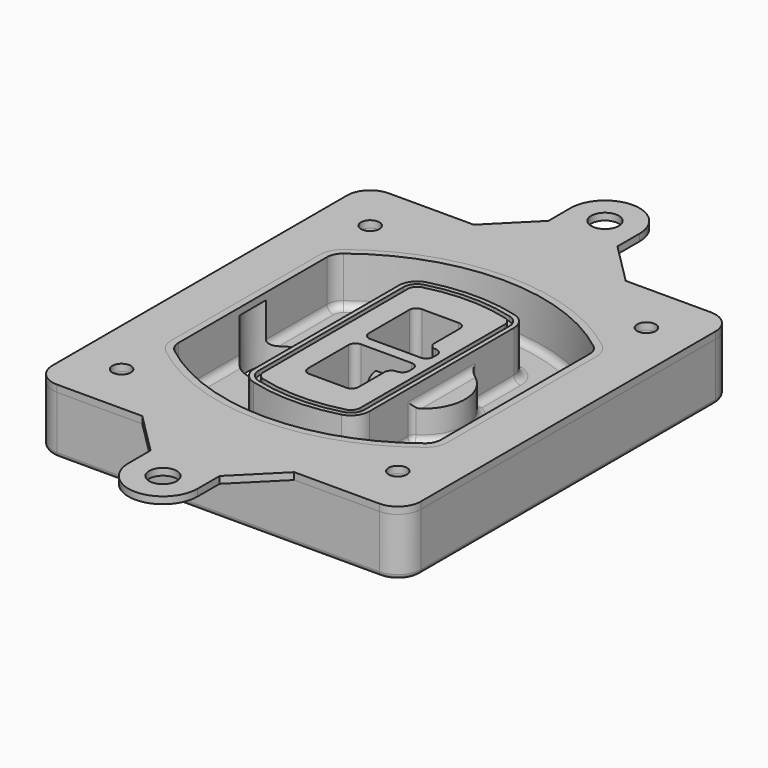
from build123d import *

# Parameters (mm, degrees)
F0_R      = 4
F1_DEPTH  = 25
F2_DEPTH  = 3
F3_DEPTH  = 18
F5_DEPTH  = 21
F6_DEPTH  = 2
F8_DEPTH  = 20
F9_DEPTH  = 16
F10_DEPTH = 25
F7_R      = 6
F7_R_2    = 4
F11_DEPTH = 6
F13_DEPTH = 9
F14_R     = 3
F15_R     = 2
F16_R     = 4
F17_DEPTH = 3
F18_D     = 12


with BuildPart() as f1:
    # F0 (on Top) → F1 (new body)
    with BuildSketch(Plane.XY):
        with BuildLine():
            ThreePointArc((-80, -80), (-77.0710678119, -87.0710678119), (-70, -90))
            Line((-70, -90), (70, -90))
            ThreePointArc((70, -90), (77.0710678119, -87.0710678119), (80, -80))
            Line((80, -80), (80, 80))
            ThreePointArc((80, 80), (77.0710678119, 87.0710678119), (70, 90))
            Line((70, 90), (-70, 90))
            ThreePointArc((-70, 90), (-77.0710678119, 87.0710678119), (-80, 80))
            Line((-80, 80), (-80, -80))
        make_face()
        with Locations((-60, -67.5)):
            Circle(F0_R, mode=Mode.SUBTRACT)
        with Locations((60, -67.5)):
            Circle(F0_R, mode=Mode.SUBTRACT)
        with Locations((-60, 67.5)):
            Circle(F0_R, mode=Mode.SUBTRACT)
        with BuildLine():
            ThreePointArc((-64, 40.2934422872), (-62.5820384798, 46.4328484224), (-58.6153846154, 51.3286200352))
            ThreePointArc((-58.6153846154, 51.3286200352), (0, 71.5), (58.6153846154, 51.3286200352))
            ThreePointArc((58.6153846154, 51.3286200352), (62.5820384798, 46.4328484224), (64, 40.2934422872))
            Line((64, 40.2934422872), (64, -40.2934422872))
            ThreePointArc((64, -40.2934422872), (62.5820384798, -46.4328484224), (58.6153846154, -51.3286200352))
            ThreePointArc((58.6153846154, -51.3286200352), (0, -71.5), (-58.6153846154, -51.3286200352))
            ThreePointArc((-58.6153846154, -51.3286200352), (-62.5820384798, -46.4328484224), (-64, -40.2934422872))
            Line((-64, -40.2934422872), (-64, 40.2934422872))
        make_face(mode=Mode.SUBTRACT)
        with Locations((60, 67.5)):
            Circle(F0_R, mode=Mode.SUBTRACT)
        with BuildLine():
            ThreePointArc((58.6153846154, 51.3286200352), (0, 71.5), (-58.6153846154, 51.3286200352))
            ThreePointArc((-58.6153846154, 51.3286200352), (-62.5820384798, 46.4328484224), (-64, 40.2934422872))
            Line((-64, 40.2934422872), (-64, -40.2934422872))
            ThreePointArc((-64, -40.2934422872), (-62.5820384798, -46.4328484224), (-58.6153846154, -51.3286200352))
            ThreePointArc((-58.6153846154, -51.3286200352), (0, -71.5), (58.6153846154, -51.3286200352))
            ThreePointArc((58.6153846154, -51.3286200352), (62.5820384798, -46.4328484224), (64, -40.2934422872))
            Line((64, -40.2934422872), (64, 40.2934422872))
            ThreePointArc((64, 40.2934422872), (62.5820384798, 46.4328484224), (58.6153846154, 51.3286200352))
        make_face()
        with BuildLine():
            Line((-60, -40.2934422872), (-60, 40.2934422872))
            ThreePointArc((-60, 40.2934422872), (-58.9871703427, 44.6787323838), (-56.1538461538, 48.1757121072))
            ThreePointArc((-56.1538461538, 48.1757121072), (0, 67.5), (56.1538461538, 48.1757121072))
            ThreePointArc((56.1538461538, 48.1757121072), (58.9871703427, 44.6787323838), (60, 40.2934422872))
            Line((60, 40.2934422872), (60, -40.2934422872))
            ThreePointArc((60, -40.2934422872), (58.9871703427, -44.6787323838), (56.1538461538, -48.1757121072))
            ThreePointArc((56.1538461538, -48.1757121072), (0, -67.5), (-56.1538461538, -48.1757121072))
            ThreePointArc((-56.1538461538, -48.1757121072), (-58.9871703427, -44.6787323838), (-60, -40.2934422872))
        make_face(mode=Mode.SUBTRACT)
        with BuildLine():
            ThreePointArc((-56.1538461538, 48.1757121072), (-58.9871703427, 44.6787323838), (-60, 40.2934422872))
            Line((-60, 40.2934422872), (-60, -40.2934422872))
            ThreePointArc((-60, -40.2934422872), (-58.9871703427, -44.6787323838), (-56.1538461538, -48.1757121072))
            ThreePointArc((-56.1538461538, -48.1757121072), (0, -67.5), (56.1538461538, -48.1757121072))
            ThreePointArc((56.1538461538, -48.1757121072), (58.9871703427, -44.6787323838), (60, -40.2934422872))
            Line((60, -40.2934422872), (60, 40.2934422872))
            ThreePointArc((60, 40.2934422872), (58.9871703427, 44.6787323838), (56.1538461538, 48.1757121072))
            ThreePointArc((56.1538461538, 48.1757121072), (0, 67.5), (-56.1538461538, 48.1757121072))
        make_face()
        with BuildLine():
            ThreePointArc((54.3076923077, 45.8110311612), (56.2910192399, 43.3631453548), (57, 40.2934422872))
            Line((57, 40.2934422872), (57, -40.2934422872))
            ThreePointArc((57, -40.2934422872), (56.2910192399, -43.3631453548), (54.3076923077, -45.8110311612))
            ThreePointArc((54.3076923077, -45.8110311612), (0, -64.5), (-54.3076923077, -45.8110311612))
            ThreePointArc((-54.3076923077, -45.8110311612), (-56.2910192399, -43.3631453548), (-57, -40.2934422872))
            Line((-57, -40.2934422872), (-57, 40.2934422872))
            ThreePointArc((-57, 40.2934422872), (-56.2910192399, 43.3631453548), (-54.3076923077, 45.8110311612))
            ThreePointArc((-54.3076923077, 45.8110311612), (0, 64.5), (54.3076923077, 45.8110311612))
        make_face(mode=Mode.SUBTRACT)
        with BuildLine():
            Line((57, -40.2934422872), (57, 40.2934422872))
            ThreePointArc((57, 40.2934422872), (56.2910192399, 43.3631453548), (54.3076923077, 45.8110311612))
            ThreePointArc((54.3076923077, 45.8110311612), (0, 64.5), (-54.3076923077, 45.8110311612))
            ThreePointArc((-54.3076923077, 45.8110311612), (-56.2910192399, 43.3631453548), (-57, 40.2934422872))
            Line((-57, 40.2934422872), (-57, -40.2934422872))
            ThreePointArc((-57, -40.2934422872), (-56.2910192399, -43.3631453548), (-54.3076923077, -45.8110311612))
            ThreePointArc((-54.3076923077, -45.8110311612), (0, -64.5), (54.3076923077, -45.8110311612))
            ThreePointArc((54.3076923077, -45.8110311612), (56.2910192399, -43.3631453548), (57, -40.2934422872))
        make_face()
    extrude(amount=-F1_DEPTH)

    # F0 (on Top) → F2 (join)
    with BuildSketch(Plane.XY):
        with BuildLine():
            ThreePointArc((-56.1538461538, 48.1757121072), (-58.9871703427, 44.6787323838), (-60, 40.2934422872))
            Line((-60, 40.2934422872), (-60, -40.2934422872))
            ThreePointArc((-60, -40.2934422872), (-58.9871703427, -44.6787323838), (-56.1538461538, -48.1757121072))
            ThreePointArc((-56.1538461538, -48.1757121072), (0, -67.5), (56.1538461538, -48.1757121072))
            ThreePointArc((56.1538461538, -48.1757121072), (58.9871703427, -44.6787323838), (60, -40.2934422872))
            Line((60, -40.2934422872), (60, 40.2934422872))
            ThreePointArc((60, 40.2934422872), (58.9871703427, 44.6787323838), (56.1538461538, 48.1757121072))
            ThreePointArc((56.1538461538, 48.1757121072), (0, 67.5), (-56.1538461538, 48.1757121072))
        make_face()
        with BuildLine():
            ThreePointArc((54.3076923077, 45.8110311612), (56.2910192399, 43.3631453548), (57, 40.2934422872))
            Line((57, 40.2934422872), (57, -40.2934422872))
            ThreePointArc((57, -40.2934422872), (56.2910192399, -43.3631453548), (54.3076923077, -45.8110311612))
            ThreePointArc((54.3076923077, -45.8110311612), (0, -64.5), (-54.3076923077, -45.8110311612))
            ThreePointArc((-54.3076923077, -45.8110311612), (-56.2910192399, -43.3631453548), (-57, -40.2934422872))
            Line((-57, -40.2934422872), (-57, 40.2934422872))
            ThreePointArc((-57, 40.2934422872), (-56.2910192399, 43.3631453548), (-54.3076923077, 45.8110311612))
            ThreePointArc((-54.3076923077, 45.8110311612), (0, 64.5), (54.3076923077, 45.8110311612))
        make_face(mode=Mode.SUBTRACT)
    extrude(amount=F2_DEPTH)

    # F0 (on Top) → F3 (cut)
    with BuildSketch(Plane.XY):
        with BuildLine():
            Line((57, -40.2934422872), (57, 40.2934422872))
            ThreePointArc((57, 40.2934422872), (56.2910192399, 43.3631453548), (54.3076923077, 45.8110311612))
            ThreePointArc((54.3076923077, 45.8110311612), (0, 64.5), (-54.3076923077, 45.8110311612))
            ThreePointArc((-54.3076923077, 45.8110311612), (-56.2910192399, 43.3631453548), (-57, 40.2934422872))
            Line((-57, 40.2934422872), (-57, -40.2934422872))
            ThreePointArc((-57, -40.2934422872), (-56.2910192399, -43.3631453548), (-54.3076923077, -45.8110311612))
            ThreePointArc((-54.3076923077, -45.8110311612), (0, -64.5), (54.3076923077, -45.8110311612))
            ThreePointArc((54.3076923077, -45.8110311612), (56.2910192399, -43.3631453548), (57, -40.2934422872))
        make_face()
    extrude(amount=-F3_DEPTH, mode=Mode.SUBTRACT)

    # F4 (on face) → F5 (join, through all)
    with BuildSketch(Plane.XY.offset(3)):
        with BuildLine():
            ThreePointArc((-25, -39.2465276821), (-23.3511545998, -44.1109737193), (-19.0842911877, -46.9702398883))
            ThreePointArc((-19.0842911877, -46.9702398883), (0, -49.5), (19.0842911877, -46.9702398883))
            ThreePointArc((19.0842911877, -46.9702398883), (23.3511545998, -44.1109737193), (25, -39.2465276821))
            Line((25, -39.2465276821), (25, 39.2465276821))
            ThreePointArc((25, 39.2465276821), (23.3511545998, 44.1109737193), (19.0842911877, 46.9702398883))
            ThreePointArc((19.0842911877, 46.9702398883), (0, 49.5), (-19.0842911877, 46.9702398883))
            ThreePointArc((-19.0842911877, 46.9702398883), (-23.3511545998, 44.1109737193), (-25, 39.2465276821))
            Line((-25, 39.2465276821), (-25, -39.2465276821))
        make_face()
        with BuildLine():
            ThreePointArc((18.5632183908, 45.0393118368), (21.7633659499, 42.89486221), (23, 39.2465276821))
            Line((23, 39.2465276821), (23, -39.2465276821))
            ThreePointArc((23, -39.2465276821), (21.7633659499, -42.89486221), (18.5632183908, -45.0393118368))
            ThreePointArc((18.5632183908, -45.0393118368), (0, -47.5), (-18.5632183908, -45.0393118368))
            ThreePointArc((-18.5632183908, -45.0393118368), (-21.7633659499, -42.89486221), (-23, -39.2465276821))
            Line((-23, -39.2465276821), (-23, 39.2465276821))
            ThreePointArc((-23, 39.2465276821), (-21.7633659499, 42.89486221), (-18.5632183908, 45.0393118368))
            ThreePointArc((-18.5632183908, 45.0393118368), (0, 47.5), (18.5632183908, 45.0393118368))
        make_face(mode=Mode.SUBTRACT)
        with BuildLine():
            Line((23, -39.2465276821), (23, 39.2465276821))
            ThreePointArc((23, 39.2465276821), (21.7633659499, 42.89486221), (18.5632183908, 45.0393118368))
            ThreePointArc((18.5632183908, 45.0393118368), (0, 47.5), (-18.5632183908, 45.0393118368))
            ThreePointArc((-18.5632183908, 45.0393118368), (-21.7633659499, 42.89486221), (-23, 39.2465276821))
            Line((-23, 39.2465276821), (-23, -39.2465276821))
            ThreePointArc((-23, -39.2465276821), (-21.7633659499, -42.89486221), (-18.5632183908, -45.0393118368))
            ThreePointArc((-18.5632183908, -45.0393118368), (0, -47.5), (18.5632183908, -45.0393118368))
            ThreePointArc((18.5632183908, -45.0393118368), (21.7633659499, -42.89486221), (23, -39.2465276821))
        make_face()
        with BuildLine():
            ThreePointArc((18.0421455939, 43.1083837852), (20.1755772999, 41.6787507007), (21, 39.2465276821))
            Line((21, 39.2465276821), (21, -39.2465276821))
            ThreePointArc((21, -39.2465276821), (20.1755772999, -41.6787507007), (18.0421455939, -43.1083837852))
            ThreePointArc((18.0421455939, -43.1083837852), (0, -45.5), (-18.0421455939, -43.1083837852))
            ThreePointArc((-18.0421455939, -43.1083837852), (-20.1755772999, -41.6787507007), (-21, -39.2465276821))
            Line((-21, -39.2465276821), (-21, 39.2465276821))
            ThreePointArc((-21, 39.2465276821), (-20.1755772999, 41.6787507007), (-18.0421455939, 43.1083837852))
            ThreePointArc((-18.0421455939, 43.1083837852), (0, 45.5), (18.0421455939, 43.1083837852))
        make_face(mode=Mode.SUBTRACT)
        with BuildLine():
            Line((21, -39.2465276821), (21, 39.2465276821))
            ThreePointArc((21, 39.2465276821), (20.1755772999, 41.6787507007), (18.0421455939, 43.1083837852))
            ThreePointArc((18.0421455939, 43.1083837852), (0, 45.5), (-18.0421455939, 43.1083837852))
            ThreePointArc((-18.0421455939, 43.1083837852), (-20.1755772999, 41.6787507007), (-21, 39.2465276821))
            Line((-21, 39.2465276821), (-21, -39.2465276821))
            ThreePointArc((-21, -39.2465276821), (-20.1755772999, -41.6787507007), (-18.0421455939, -43.1083837852))
            ThreePointArc((-18.0421455939, -43.1083837852), (0, -45.5), (18.0421455939, -43.1083837852))
            ThreePointArc((18.0421455939, -43.1083837852), (20.1755772999, -41.6787507007), (21, -39.2465276821))
        make_face()
        with BuildLine():
            Line((-8, -2.5), (14, -2.5))
            ThreePointArc((14, -2.5), (16.1213203436, -3.3786796564), (17, -5.5))
            Line((17, -5.5), (17, -7.5))
            ThreePointArc((17, -7.5), (16.1213203436, -9.6213203436), (14, -10.5))
            ThreePointArc((14, -10.5), (11.8786796564, -11.3786796564), (11, -13.5))
            Line((11, -13.5), (11, -27.5))
            ThreePointArc((11, -27.5), (10.1213203436, -29.6213203436), (8, -30.5))
            Line((8, -30.5), (-8, -30.5))
            ThreePointArc((-8, -30.5), (-10.1213203436, -29.6213203436), (-11, -27.5))
            Line((-11, -27.5), (-11, -5.5))
            ThreePointArc((-11, -5.5), (-10.1213203436, -3.3786796564), (-8, -2.5))
        make_face(mode=Mode.SUBTRACT)
        with BuildLine():
            ThreePointArc((-8, 2.5), (-10.1213203436, 3.3786796564), (-11, 5.5))
            Line((-11, 5.5), (-11, 27.5))
            ThreePointArc((-11, 27.5), (-10.1213203436, 29.6213203436), (-8, 30.5))
            Line((-8, 30.5), (8, 30.5))
            ThreePointArc((8, 30.5), (10.1213203436, 29.6213203436), (11, 27.5))
            Line((11, 27.5), (11, 13.5))
            ThreePointArc((11, 13.5), (11.8786796564, 11.3786796564), (14, 10.5))
            ThreePointArc((14, 10.5), (16.1213203436, 9.6213203436), (17, 7.5))
            Line((17, 7.5), (17, 5.5))
            ThreePointArc((17, 5.5), (16.1213203436, 3.3786796564), (14, 2.5))
            Line((14, 2.5), (-8, 2.5))
        make_face(mode=Mode.SUBTRACT)
    extrude(amount=-F5_DEPTH)

    # F4 (on face) → F6 (cut)
    with BuildSketch(Plane.XY.offset(3)):
        with BuildLine():
            Line((23, -39.2465276821), (23, 39.2465276821))
            ThreePointArc((23, 39.2465276821), (21.7633659499, 42.89486221), (18.5632183908, 45.0393118368))
            ThreePointArc((18.5632183908, 45.0393118368), (0, 47.5), (-18.5632183908, 45.0393118368))
            ThreePointArc((-18.5632183908, 45.0393118368), (-21.7633659499, 42.89486221), (-23, 39.2465276821))
            Line((-23, 39.2465276821), (-23, -39.2465276821))
            ThreePointArc((-23, -39.2465276821), (-21.7633659499, -42.89486221), (-18.5632183908, -45.0393118368))
            ThreePointArc((-18.5632183908, -45.0393118368), (0, -47.5), (18.5632183908, -45.0393118368))
            ThreePointArc((18.5632183908, -45.0393118368), (21.7633659499, -42.89486221), (23, -39.2465276821))
        make_face()
        with BuildLine():
            ThreePointArc((18.0421455939, 43.1083837852), (20.1755772999, 41.6787507007), (21, 39.2465276821))
            Line((21, 39.2465276821), (21, -39.2465276821))
            ThreePointArc((21, -39.2465276821), (20.1755772999, -41.6787507007), (18.0421455939, -43.1083837852))
            ThreePointArc((18.0421455939, -43.1083837852), (0, -45.5), (-18.0421455939, -43.1083837852))
            ThreePointArc((-18.0421455939, -43.1083837852), (-20.1755772999, -41.6787507007), (-21, -39.2465276821))
            Line((-21, -39.2465276821), (-21, 39.2465276821))
            ThreePointArc((-21, 39.2465276821), (-20.1755772999, 41.6787507007), (-18.0421455939, 43.1083837852))
            ThreePointArc((-18.0421455939, 43.1083837852), (0, 45.5), (18.0421455939, 43.1083837852))
        make_face(mode=Mode.SUBTRACT)
    extrude(amount=-F6_DEPTH, mode=Mode.SUBTRACT)

    # F7 (on face) → F8 (join)
    with BuildSketch(Plane(origin=(0, 0, -25), x_dir=(1, 0, 0), z_dir=(0, 0, -1))):
        with BuildLine():
            ThreePointArc((3.28842436, 0), (16.7567035675, 13.4682792075), (30.224982775, 0))
            Line((30.224982775, 0), (35.224982775, 0))
            ThreePointArc((35.224982775, 0), (16.7567035675, 18.4682792075), (-1.71157564, 0))
            Line((-1.71157564, 0), (3.28842436, 0))
        make_face()
        with BuildLine():
            Line((3.28842436, 0), (30.224982775, 0))
            ThreePointArc((30.224982775, 0), (16.7567035675, 13.4682792075), (3.28842436, 0))
        make_face()
        with BuildLine():
            ThreePointArc((3.28842436, 0), (16.7567035675, -13.4682792075), (30.224982775, 0))
            Line((30.224982775, 0), (3.28842436, 0))
        make_face()
        with BuildLine():
            Line((35.224982775, 0), (30.224982775, 0))
            ThreePointArc((30.224982775, 0), (16.7567035675, -13.4682792075), (3.28842436, 0))
            Line((3.28842436, 0), (-1.71157564, 0))
            ThreePointArc((-1.71157564, 0), (16.7567035675, -18.4682792075), (35.224982775, 0))
        make_face()
    extrude(amount=-F8_DEPTH)

    # F7 (on face) → F9 (cut)
    with BuildSketch(Plane(origin=(0, 0, -25), x_dir=(1, 0, 0), z_dir=(0, 0, -1))):
        with BuildLine():
            Line((3.28842436, 0), (30.224982775, 0))
            ThreePointArc((30.224982775, 0), (16.7567035675, 13.4682792075), (3.28842436, 0))
        make_face()
        with BuildLine():
            ThreePointArc((3.28842436, 0), (16.7567035675, -13.4682792075), (30.224982775, 0))
            Line((30.224982775, 0), (3.28842436, 0))
        make_face()
    extrude(amount=-F9_DEPTH, mode=Mode.SUBTRACT)

    # F7 (on face) → F10 (cut)
    with BuildSketch(Plane(origin=(0, 0, -25), x_dir=(1, 0, 0), z_dir=(0, 0, -1))):
        with BuildLine():
            Line((-59.0318229325, 0), (-32.0952645175, 0))
            ThreePointArc((-32.0952645175, 0), (-45.563543725, 13.4682792075), (-59.0318229325, 0))
        make_face()
        with BuildLine():
            ThreePointArc((-59.0318229325, 0), (-45.563543725, -13.4682792075), (-32.0952645175, 0))
            Line((-32.0952645175, 0), (-59.0318229325, 0))
        make_face()
    extrude(amount=-F10_DEPTH, mode=Mode.SUBTRACT)

    # F7 (on face) → F11 (cut)
    with BuildSketch(Plane(origin=(0, 0, -25), x_dir=(1, 0, 0), z_dir=(0, 0, -1))):
        with Locations((60, -67.5)):
            Circle(F7_R)
        with Locations((60, -67.5)):
            Circle(F7_R_2, mode=Mode.SUBTRACT)
        with Locations((-60, -67.5)):
            Circle(F7_R)
        with Locations((-60, -67.5)):
            Circle(F7_R_2, mode=Mode.SUBTRACT)
        with Locations((-60, 67.5)):
            Circle(F7_R)
        with Locations((-60, 67.5)):
            Circle(F7_R_2, mode=Mode.SUBTRACT)
        with Locations((60, 67.5)):
            Circle(F7_R)
        with Locations((60, 67.5)):
            Circle(F7_R_2, mode=Mode.SUBTRACT)
    extrude(amount=-F11_DEPTH, mode=Mode.SUBTRACT)

    # F12 (on face) → F13 (cut, through all)
    with BuildSketch(Plane(origin=(0, 0, -9), x_dir=(1, 0, 0), z_dir=(0, 0, -1))):
        with BuildLine():
            Line((11, 13.5), (11, 17.5481537753))
            ThreePointArc((11, 17.5481537753), (2.5696536419, 11.8239143813), (-1.5415842455, 2.5))
            Line((-1.5415842455, 2.5), (3.5224848595, 2.5))
            ThreePointArc((3.5224848595, 2.5), (6.1857188154, 8.3455872281), (11.2536447004, 12.2927168648))
            ThreePointArc((11.2536447004, 12.2927168648), (11.0640958889, 12.8831798879), (11, 13.5))
        make_face()
        with BuildLine():
            ThreePointArc((11.2536447004, -12.2927168648), (6.1857188154, -8.3455872281), (3.5224848595, -2.5))
            Line((3.5224848595, -2.5), (-1.5415842455, -2.5))
            ThreePointArc((-1.5415842455, -2.5), (2.5696536419, -11.8239143813), (11, -17.5481537753))
            Line((11, -17.5481537753), (11, -13.5))
            ThreePointArc((11, -13.5), (11.0640958889, -12.8831798879), (11.2536447004, -12.2927168648))
        make_face()
        with BuildLine():
            ThreePointArc((11.2536447004, 12.2927168648), (6.1857188154, 8.3455872281), (3.5224848595, 2.5))
            Line((3.5224848595, 2.5), (14, 2.5))
            ThreePointArc((14, 2.5), (16.1213203436, 3.3786796564), (17, 5.5))
            Line((17, 5.5), (17, 7.5))
            ThreePointArc((17, 7.5), (16.1213203436, 9.6213203436), (14, 10.5))
            ThreePointArc((14, 10.5), (12.3601599782, 10.9878446101), (11.2536447004, 12.2927168648))
        make_face()
        with BuildLine():
            Line((14, -2.5), (3.5224848595, -2.5))
            ThreePointArc((3.5224848595, -2.5), (6.1857188154, -8.3455872281), (11.2536447004, -12.2927168648))
            ThreePointArc((11.2536447004, -12.2927168648), (12.3601599782, -10.9878446101), (14, -10.5))
            ThreePointArc((14, -10.5), (16.1213203436, -9.6213203436), (17, -7.5))
            Line((17, -7.5), (17, -5.5))
            ThreePointArc((17, -5.5), (16.1213203436, -3.3786796564), (14, -2.5))
        make_face()
    extrude(amount=F13_DEPTH, mode=Mode.SUBTRACT)

    # F14
    f14_edges = [f1.edges().sort_by_distance(p)[0] for p in [
        (-57, -23.703476, -18),
        (-57, 23.703476, -18),
        (25, 0, -5),
        (25, 16.526506, -11.5),
        (25, -16.526506, -11.5),
        (25, -27.886517, -18),
        (35.224983, 0, -18),
    ]]
    fillet(f14_edges, radius=F14_R)

    # F15
    f15_edges = [f1.edges().sort_by_distance(p)[0] for p in [
        (0, -90, -25),
    ]]
    fillet(f15_edges, radius=F15_R)


with BuildPart() as f17:
    # F16 (on face) → F17 (new body, through all)
    with BuildSketch(Plane.XY):
        with BuildLine():
            Line((33, 90), (0, 90))
            Line((0, 90), (-33, 90))
            Line((-33, 90), (-70, 90))
            ThreePointArc((-70, 90), (-77.0710678119, 87.0710678119), (-80, 80))
            Line((-80, 80), (-80, 0))
            Line((-80, 0), (-60, 0))
            Line((-60, 0), (-60, 40.2934422872))
            ThreePointArc((-60, 40.2934422872), (-58.9871703427, 44.6787323838), (-56.1538461538, 48.1757121072))
            ThreePointArc((-56.1538461538, 48.1757121072), (0, 67.5), (56.1538461538, 48.1757121072))
            ThreePointArc((56.1538461538, 48.1757121072), (58.9871703427, 44.6787323838), (60, 40.2934422872))
            Line((60, 40.2934422872), (60, 0))
            Line((60, 0), (80, 0))
            Line((80, 0), (80, 80))
            ThreePointArc((80, 80), (77.0710678119, 87.0710678119), (70, 90))
            Line((70, 90), (33, 90))
        make_face()
        with Locations((-60, 67.5)):
            Circle(F16_R, mode=Mode.SUBTRACT)
        with Locations((60, 67.5)):
            Circle(F16_R, mode=Mode.SUBTRACT)
        with BuildLine():
            Line((80, -80), (80, 0))
            Line((80, 0), (60, 0))
            Line((60, 0), (60, -40.2934422872))
            ThreePointArc((60, -40.2934422872), (58.9871703427, -44.6787323838), (56.1538461538, -48.1757121072))
            ThreePointArc((56.1538461538, -48.1757121072), (0, -67.5), (-56.1538461538, -48.1757121072))
            ThreePointArc((-56.1538461538, -48.1757121072), (-58.9871703427, -44.6787323838), (-60, -40.2934422872))
            Line((-60, -40.2934422872), (-60, 0))
            Line((-60, 0), (-80, 0))
            Line((-80, 0), (-80, -80))
            ThreePointArc((-80, -80), (-77.0710678119, -87.0710678119), (-70, -90))
            Line((-70, -90), (-33, -90))
            Line((-33, -90), (0, -90))
            Line((0, -90), (33, -90))
            Line((33, -90), (70, -90))
            ThreePointArc((70, -90), (77.0710678119, -87.0710678119), (80, -80))
        make_face()
        with Locations((-60, -67.5)):
            Circle(F16_R, mode=Mode.SUBTRACT)
        with Locations((60, -67.5)):
            Circle(F16_R, mode=Mode.SUBTRACT)
        with BuildLine():
            Line((-33, 90), (0, 90))
            Line((0, 90), (33, 90))
            Line((33, 90), (15, 108))
            Line((15, 108), (15, 120))
            ThreePointArc((15, 120), (0, 135), (-15, 120))
            Line((-15, 120), (-15, 108))
            Line((-15, 108), (-33, 90))
        make_face()
        with BuildLine():
            ThreePointArc((6, 120), (4.2426406871, 115.7573593129), (0, 114))
            ThreePointArc((0, 114), (-4.2426406871, 124.2426406871), (6, 120))
        make_face(mode=Mode.SUBTRACT)
        with BuildLine():
            Line((15, -108), (33, -90))
            Line((33, -90), (0, -90))
            Line((0, -90), (-33, -90))
            Line((-33, -90), (-15, -108))
            Line((-15, -108), (-15, -120))
            ThreePointArc((-15, -120), (0, -135), (15, -120))
            Line((15, -120), (15, -108))
        make_face()
        with BuildLine():
            ThreePointArc((6, -120), (-4.2426406871, -124.2426406871), (0, -114))
            ThreePointArc((0, -114), (4.2426406871, -115.7573593129), (6, -120))
        make_face(mode=Mode.SUBTRACT)
        with BuildLine():
            ThreePointArc((0, 114), (4.2426406871, 115.7573593129), (6, 120))
            ThreePointArc((6, 120), (-4.2426406871, 124.2426406871), (0, 114))
        make_face()
        with BuildLine():
            ThreePointArc((0, -114), (-4.2426406871, -124.2426406871), (6, -120))
            ThreePointArc((6, -120), (4.2426406871, -115.7573593129), (0, -114))
        make_face()
    extrude(amount=F17_DEPTH)

    # F18 (through all)
    with Locations(Plane(origin=(0, 0, 0), x_dir=(1, 0, 0), z_dir=(0, 0, -1))):
        with Locations((0, -120), (0, 120)):
            Hole(F18_D / 2)


solid = Compound([f1.part, f17.part])
